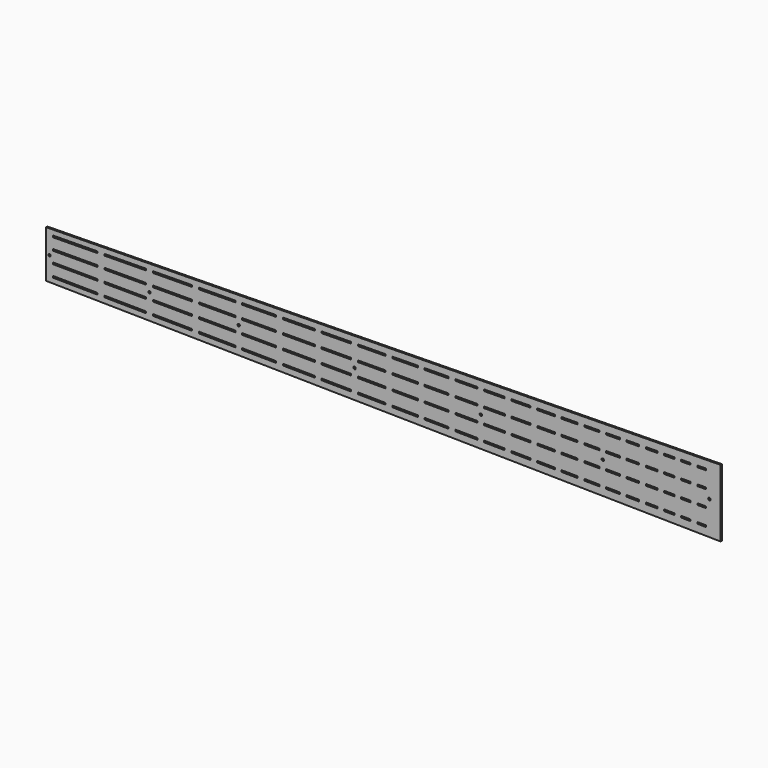
from build123d import *

# Parameters (mm, degrees)
F2_DEPTH = 1.524
F4_DEPTH = 1.525
F5_R     = 1.1303
F6_DEPTH = 979
F7_DEPTH = 1.525


# Not quite as in the source:
# - an extrude ends at something that could not be found from the text; its depth is read off the source's solid


with BuildPart() as f2:
    # F1 (on Front) → F2 (new body)
    with BuildSketch(Plane.XZ):
        Polygon((0, 44.45), (0, 0), (635, -9.525), (635, 53.975), align=None)
    extrude(amount=F2_DEPTH)

    # F0 (on Front) → F4 (cut, through all)
    with BuildSketch(Plane.XZ):
        Polygon((6.3580304305, 6.2480541955), (6.3496125138, 5.4861006938), (6.341194597, 4.7241471921), (48.4590379481, 4.2588373038), (48.4674558648, 5.0207908055), (48.4758737815, 5.7827443071), align=None)
        Polygon((54.8254862953, 5.7125950009), (54.8170683786, 4.9506414993), (54.8086504618, 4.1886879976), (94.2054562647, 3.7534396124), (94.2138741814, 4.515393114), (94.2222920981, 5.2773466157), align=None)
        Polygon((100.5719046119, 5.2071973095), (100.5634866952, 4.4452438078), (100.5550687784, 3.6832903062), (137.385412, 3.2763957093), (137.3938299168, 4.0383492109), (137.4022478336, 4.8003027126), align=None)
        Polygon((143.7518603473, 4.7301534064), (143.7434424306, 3.9681999047), (143.7350245139, 3.2062464031), (178.1336185335, 2.8262173069), (178.1420364502, 3.5881708085), (178.150454367, 4.3501243102), align=None)
        Polygon((184.5000668807, 4.279975004), (184.491648964, 3.5180215023), (184.4832310472, 2.7560680007), (216.6098321156, 2.4011394486), (216.6182500324, 3.1630929503), (216.6266679491, 3.9250464519), align=None)
        Polygon((222.9762804629, 3.8548971457), (222.9678625461, 3.0929436441), (222.9594446294, 2.3309901424), (252.9185419701, 2.0000077576), (252.9269598868, 2.7619612592), (252.9353778036, 3.5239147609), align=None)
        Polygon((259.2849903173, 3.4537654547), (259.2765724006, 2.691811953), (259.2681544838, 1.9298584514), (287.1901437394, 1.6213816475), (287.1985616562, 2.3833351492), (287.2069795729, 3.1452886508), align=None)
        Polygon((293.5565920867, 3.0751393446), (293.5481741699, 2.313185843), (293.5397562532, 1.5512323413), (319.5377621202, 1.2640113384), (319.5461800369, 2.0259648401), (319.5545979537, 2.7879183417), align=None)
        Polygon((325.9042104674, 2.7177690355), (325.8957925507, 1.9558155339), (325.887374634, 1.1938620322), (350.0702040724, 0.9266947518), (350.0786219892, 1.6886482534), (350.0870399059, 2.4506017551), align=None)
        Polygon((356.4366524197, 2.3804524489), (356.4282345029, 1.6184989472), (356.4198165862, 0.8565454456), (378.8893681778, 0.6083061315), (378.8977860945, 1.3702596332), (378.9062040113, 2.1322131349), align=None)
        Polygon((385.255816525, 2.0620638286), (385.2473986083, 1.300110327), (385.2389806915, 0.5381568253), (406.0902446394, 0.3077960441), (406.0986625561, 1.0697495457), (406.1070804729, 1.8317030474), align=None)
        Polygon((412.4566929866, 1.7615537412), (412.4482750699, 0.9996002395), (412.4398571532, 0.2376467379), (431.7652330186, 0.0241436767), (431.7736509354, 0.7860971784), (431.7820688521, 1.54805068), align=None)
        Polygon((438.1316813659, 1.4779013738), (438.1232634491, 0.7159478722), (438.1148455324, -0.0460056295), (455.998960951, -0.2435859206), (456.0073788678, 0.5183675811), (456.0157967845, 1.2803210827), align=None)
        Polygon((462.3654092983, 1.2101717765), (462.3569913815, 0.4482182749), (462.3485734648, -0.3137352268), (478.872601883, -0.4962895364), (478.8810197997, 0.2656639652), (478.8894377165, 1.0276174669), align=None)
        Polygon((485.2390502302, 0.9574681607), (485.2306323135, 0.195514659), (485.2222143967, -0.5664388426), (500.462147977, -0.7348067178), (500.4705658938, 0.0271467838), (500.4789838105, 0.7891002855), align=None)
        Polygon((506.8285963243, 0.7189509793), (506.8201784075, -0.0430025224), (506.8117604908, -0.804956024), (520.8401372066, -0.9599388504), (520.8485551233, -0.1979853487), (520.8569730401, 0.5639681529), align=None)
        Polygon((527.2065855538, 0.4938188467), (527.1981676371, -0.268134655), (527.1897497203, -1.0300881566), (540.0739262612, -1.172430078), (540.0823441779, -0.4104765763), (540.0907620946, 0.3514769253), align=None)
        Polygon((546.4403746084, 0.2813276191), (546.4319566917, -0.4806258825), (546.4235387749, -1.2425793842), (558.2291447357, -1.3730054638), (558.2375626524, -0.6110519622), (558.2459805692, 0.1509015395), align=None)
        Polygon((564.5955930829, 0.0807522333), (564.5871751662, -0.6812012684), (564.5787572494, -1.44315477), (575.3645138467, -1.5623137487), (575.3729317635, -0.8003602471), (575.3813496802, -0.0384067454), align=None)
        Polygon((581.730962194, -0.1085560516), (581.7225442772, -0.8705095533), (581.7141263605, -1.6324630549), (591.5387548107, -1.7410036734), (591.5471727275, -0.9790501718), (591.5555906442, -0.2170966701), align=None)
        Polygon((597.905203158, -0.2872459763), (597.8967852412, -1.049199478), (597.8883673245, -1.8111529796), (606.8045440132, -1.9096571966), (606.81296193, -1.1477036949), (606.8213798467, -0.3857501933), align=None)
        Polygon((613.1709923605, -0.4558994995), (613.1625744437, -1.2178530011), (613.154156527, -1.9798065028), (621.2145578395, -2.0688562768), (621.2229757563, -1.3069027752), (621.231393673, -0.5449492735), align=None)
        Polygon((6.3527629194, 17.4073617316), (6.3499569471, 16.6453668979), (6.3471509749, 15.8833720643), (48.4672789994, 15.7282687682), (48.4700849717, 16.4902636018), (48.4728909439, 17.2522584355), align=None)
        Polygon((54.8228478911, 17.2288753334), (54.8200419188, 16.4668804998), (54.8172359466, 15.7048856661), (94.2161788208, 15.559802871), (94.218984793, 16.3217977047), (94.2217907653, 17.0837925383), align=None)
        Polygon((100.5717477124, 17.0604094363), (100.5689417402, 16.2984146026), (100.5661357679, 15.5364197689), (137.3984768438, 15.4007882367), (137.401282816, 16.1627830703), (137.4040887883, 16.924777904), align=None)
        Polygon((143.7540457354, 16.9013948019), (143.7512397632, 16.1393999682), (143.7484337909, 15.3774051346), (178.148893755, 15.2507287692), (178.1516997272, 16.0127236028), (178.1545056995, 16.7747184365), align=None)
        Polygon((184.5044626466, 16.7513353344), (184.5016566744, 15.9893405008), (184.4988507021, 15.2273456671), (216.6271944712, 15.1090361498), (216.6300004434, 15.8710309834), (216.6328064157, 16.6330258171), align=None)
        Polygon((222.9827633628, 16.609642715), (222.9799573906, 15.8476478814), (222.9771514183, 15.0856530477), (252.9378738839, 14.9753255861), (252.9406798562, 15.7373204197), (252.9434858284, 16.4993152534), align=None)
        Polygon((259.2934427755, 16.4759321513), (259.2906368033, 15.7139373177), (259.2878308311, 14.951942484), (287.211334709, 14.8491168827), (287.2141406813, 15.6111117164), (287.2169466535, 16.37310655), align=None)
        Polygon((293.5669036007, 16.349723448), (293.5640976284, 15.5877286143), (293.5612916562, 14.8257337807), (319.5607077795, 14.7299934464), (319.5635137518, 15.49198828), (319.566319724, 16.2539831137), align=None)
        Polygon((325.9162766711, 16.2306000116), (325.9134706989, 15.468605178), (325.9106647266, 14.7066103443), (350.0948059576, 14.6175545842), (350.0976119298, 15.3795494178), (350.1004179021, 16.1415442515), align=None)
        Polygon((356.4503748492, 16.1181611494), (356.447568877, 15.3561663157), (356.4447629047, 14.5941714821), (378.9155333524, 14.5114250441), (378.9183393246, 15.2734198777), (378.9211452969, 16.0354147114), align=None)
        Polygon((385.271102244, 16.0120316093), (385.2682962718, 15.2500367757), (385.2654902995, 14.488041942), (406.1178853198, 14.4112550149), (406.120691292, 15.1732498486), (406.1234972643, 15.9352446822), align=None)
        Polygon((412.4734542114, 15.9118615802), (412.4706482392, 15.1498667465), (412.4678422669, 14.3878719129), (431.7942664333, 14.3167042258), (431.7970724056, 15.0786990595), (431.7998783778, 15.8406938931), align=None)
        Polygon((438.1498353249, 15.817310791), (438.1470293527, 15.0553159574), (438.1442233804, 14.2933211237), (456.0293089191, 14.2274610267), (456.0321148914, 14.9894558604), (456.0349208636, 15.751450694), align=None)
        Polygon((462.3848778108, 15.728067592), (462.3820718385, 14.9660727583), (462.3792658663, 14.2040779246), (478.9041906269, 14.1432264881), (478.9069965991, 14.9052213217), (478.9098025714, 15.6672161554), align=None)
        Polygon((485.2597595185, 15.6438330533), (485.2569535463, 14.8818382197), (485.254147574, 14.119843386), (500.4949078413, 14.063720761), (500.4977138136, 14.8257155946), (500.5005197858, 15.5877104283), align=None)
        Polygon((506.850476733, 15.5643273262), (506.8476707607, 14.8023324925), (506.8448647885, 14.0403376589), (520.8740024706, 13.9886767168), (520.8768084428, 14.7506715504), (520.8796144151, 15.5126663841), align=None)
        Polygon((527.2295713622, 15.489283282), (527.22676539, 14.7272884483), (527.2239594177, 13.9652936147), (540.1088348579, 13.9178463076), (540.1116408302, 14.6798411412), (540.1144468024, 15.4418359749), align=None)
        Polygon((546.4644037496, 15.4184528728), (546.4615977773, 14.6564580392), (546.4587918051, 13.8944632055), (558.2650381585, 13.8509878456), (558.2678441307, 14.6129826793), (558.270650103, 15.3749775129), align=None)
        Polygon((564.6206070501, 15.3515944109), (564.6178010778, 14.5895995772), (564.6149951056, 13.8276047435), (575.4013367739, 13.787885084), (575.4041427462, 14.5498799176), (575.4069487184, 15.3118747513), align=None)
        Polygon((581.7569056656, 15.2884916492), (581.7540996933, 14.5264968156), (581.7512937211, 13.7645019819), (591.5764551063, 13.7283217758), (591.5792610785, 14.4903166094), (591.5820670508, 15.2523114431), align=None)
        Polygon((597.9320239979, 15.228928341), (597.9292180256, 14.4669335073), (597.9264120534, 13.7049386737), (606.8430723982, 13.6721039347), (606.8458783705, 14.4340987684), (606.8486843427, 15.196093602), align=None)
        Polygon((613.1986412899, 15.1727104999), (613.1958353176, 14.4107156663), (613.1930293454, 13.6487208326), (621.2538678927, 13.6190375746), (621.2566738649, 14.3810324083), (621.2594798372, 15.1430272419), align=None)
        Polygon((6.3471509749, 28.5666279357), (6.3499569471, 27.8046331021), (6.3527629194, 27.0426382684), (48.4728909439, 27.1977415645), (48.4700849717, 27.9597363982), (48.4672789994, 28.7217312318), align=None)
        Polygon((54.8172359466, 28.7451143339), (54.8200419188, 27.9831195002), (54.8228478911, 27.2211246666), (94.2217907653, 27.3662074617), (94.218984793, 28.1282022953), (94.2161788208, 28.890197129), align=None)
        Polygon((100.5661357679, 28.9135802311), (100.5689417402, 28.1515853974), (100.5717477124, 27.3895905637), (137.4040887883, 27.525222096), (137.401282816, 28.2872169297), (137.3984768438, 29.0492117633), align=None)
        Polygon((143.7484337909, 29.0725948654), (143.7512397632, 28.3106000318), (143.7540457354, 27.5486051981), (178.1545056995, 27.6752815635), (178.1516997272, 28.4372763972), (178.148893755, 29.1992712308), align=None)
        Polygon((184.4988507021, 29.2226543329), (184.5016566744, 28.4606594992), (184.5044626466, 27.6986646656), (216.6328064157, 27.8169741829), (216.6300004434, 28.5789690166), (216.6271944712, 29.3409638502), align=None)
        Polygon((222.9771514183, 29.3643469523), (222.9799573906, 28.6023521186), (222.9827633628, 27.840357285), (252.9434858284, 27.9506847466), (252.9406798562, 28.7126795803), (252.9378738839, 29.4746744139), align=None)
        Polygon((259.2878308311, 29.498057516), (259.2906368033, 28.7360626823), (259.2934427755, 27.9740678487), (287.2169466535, 28.07689345), (287.2141406813, 28.8388882836), (287.211334709, 29.6008831173), align=None)
        Polygon((293.5612916562, 29.6242662193), (293.5640976284, 28.8622713857), (293.5669036007, 28.100276552), (319.566319724, 28.1960168863), (319.5635137518, 28.95801172), (319.5607077795, 29.7200065536), align=None)
        Polygon((325.9106647266, 29.7433896557), (325.9134706989, 28.981394822), (325.9162766711, 28.2193999884), (350.1004179021, 28.3084557485), (350.0976119298, 29.0704505822), (350.0948059576, 29.8324454158), align=None)
        Polygon((356.4447629047, 29.8558285179), (356.447568877, 29.0938336843), (356.4503748492, 28.3318388506), (378.9211452969, 28.4145852886), (378.9183393246, 29.1765801223), (378.9155333524, 29.9385749559), align=None)
        Polygon((385.2654902995, 29.961958058), (385.2682962718, 29.1999632243), (385.271102244, 28.4379683907), (406.1234972643, 28.5147553178), (406.120691292, 29.2767501514), (406.1178853198, 30.0387449851), align=None)
        Polygon((412.4678422669, 30.0621280871), (412.4706482392, 29.3001332535), (412.4734542114, 28.5381384198), (431.7998783778, 28.6093061069), (431.7970724056, 29.3713009405), (431.7942664333, 30.1332957742), align=None)
        Polygon((438.1442233804, 30.1566788763), (438.1470293527, 29.3946840426), (438.1498353249, 28.632689209), (456.0349208636, 28.698549306), (456.0321148914, 29.4605441396), (456.0293089191, 30.2225389733), align=None)
        Polygon((462.3792658663, 30.2459220754), (462.3820718385, 29.4839272417), (462.3848778108, 28.721932408), (478.9098025714, 28.7827838446), (478.9069965991, 29.5447786783), (478.9041906269, 30.3067735119), align=None)
        Polygon((485.254147574, 30.330156614), (485.2569535463, 29.5681617803), (485.2597595185, 28.8061669467), (500.5005197858, 28.8622895717), (500.4977138136, 29.6242844054), (500.4949078413, 30.386279239), align=None)
        Polygon((506.8448647885, 30.4096623411), (506.8476707607, 29.6476675075), (506.850476733, 28.8856726738), (520.8796144151, 28.9373336159), (520.8768084428, 29.6993284496), (520.8740024706, 30.4613232832), align=None)
        Polygon((527.2239594177, 30.4847063853), (527.22676539, 29.7227115517), (527.2295713622, 28.960716718), (540.1144468024, 29.0081640251), (540.1116408302, 29.7701588588), (540.1088348579, 30.5321536924), align=None)
        Polygon((546.4587918051, 30.5555367945), (546.4615977773, 29.7935419608), (546.4644037496, 29.0315471272), (558.270650103, 29.0750224871), (558.2678441307, 29.8370173207), (558.2650381585, 30.5990121544), align=None)
        Polygon((564.6149951056, 30.6223952565), (564.6178010778, 29.8604004228), (564.6206070501, 29.0984055891), (575.4069487184, 29.1381252487), (575.4041427462, 29.9001200824), (575.4013367739, 30.662114916), align=None)
        Polygon((581.7512937211, 30.6854980181), (581.7540996933, 29.9235031844), (581.7569056656, 29.1615083508), (591.5820670508, 29.1976885569), (591.5792610785, 29.9596833906), (591.5764551063, 30.7216782242), align=None)
        Polygon((597.9264120534, 30.7450613263), (597.9292180256, 29.9830664927), (597.9320239979, 29.221071659), (606.8486843427, 29.253906398), (606.8458783705, 30.0159012316), (606.8430723982, 30.7778960653), align=None)
        Polygon((613.1930293454, 30.8012791674), (613.1958353176, 30.0392843337), (613.1986412899, 29.2772895001), (621.2594798372, 29.3069727581), (621.2566738649, 30.0689675917), (621.2538678927, 30.8309624254), align=None)
        Polygon((6.341194597, 39.7258528079), (6.3496125138, 38.9638993062), (6.3580304305, 38.2019458046), (48.4758737815, 38.6672556929), (48.4674558648, 39.4292091945), (48.4590379481, 40.1911626962), align=None)
        Polygon((54.8086504618, 40.2613120024), (54.8170683786, 39.4993585007), (54.8254862953, 38.7374049991), (94.2222920981, 39.1726533843), (94.2138741814, 39.934606886), (94.2054562647, 40.6965603876), align=None)
        Polygon((100.5550687784, 40.7667096938), (100.5634866952, 40.0047561922), (100.5719046119, 39.2428026905), (137.4022478336, 39.6496972874), (137.3938299168, 40.4116507891), (137.385412, 41.1736042907), align=None)
        Polygon((143.7350245139, 41.2437535969), (143.7434424306, 40.4818000953), (143.7518603473, 39.7198465936), (178.150454367, 40.0998756898), (178.1420364502, 40.8618291915), (178.1336185335, 41.6237826931), align=None)
        Polygon((184.4832310472, 41.6939319993), (184.491648964, 40.9319784977), (184.5000668807, 40.170024996), (216.6266679491, 40.5249535481), (216.6182500324, 41.2869070497), (216.6098321156, 42.0488605514), align=None)
        Polygon((222.9594446294, 42.1190098576), (222.9678625461, 41.3570563559), (222.9762804629, 40.5951028543), (252.9353778036, 40.9260852391), (252.9269598868, 41.6880387408), (252.9185419701, 42.4499922424), align=None)
        Polygon((259.2681544838, 42.5201415486), (259.2765724006, 41.758188047), (259.2849903173, 40.9962345453), (287.2069795729, 41.3047113492), (287.1985616562, 42.0666648508), (287.1901437394, 42.8286183525), align=None)
        Polygon((293.5397562532, 42.8987676587), (293.5481741699, 42.136814157), (293.5565920867, 41.3748606554), (319.5545979537, 41.6620816583), (319.5461800369, 42.4240351599), (319.5377621202, 43.1859886616), align=None)
        Polygon((325.887374634, 43.2561379678), (325.8957925507, 42.4941844661), (325.9042104674, 41.7322309645), (350.0870399059, 41.9993982449), (350.0786219892, 42.7613517466), (350.0702040724, 43.5233052482), align=None)
        Polygon((356.4198165862, 43.5934545544), (356.4282345029, 42.8315010528), (356.4366524197, 42.0695475511), (378.9062040113, 42.3177868652), (378.8977860945, 43.0797403668), (378.8893681778, 43.8416938685), align=None)
        Polygon((385.2389806915, 43.9118431747), (385.2473986083, 43.149889673), (385.255816525, 42.3879361714), (406.1070804729, 42.6182969526), (406.0986625561, 43.3802504543), (406.0902446394, 44.1422039559), align=None)
        Polygon((412.4398571532, 44.2123532621), (412.4482750699, 43.4503997605), (412.4566929866, 42.6884462588), (431.7820688521, 42.90194932), (431.7736509354, 43.6639028216), (431.7652330186, 44.4258563233), align=None)
        Polygon((438.1148455324, 44.4960056295), (438.1232634491, 43.7340521278), (438.1316813659, 42.9720986262), (456.0157967845, 43.1696789173), (456.0073788678, 43.9316324189), (455.998960951, 44.6935859206), align=None)
        Polygon((462.3485734648, 44.7637352268), (462.3569913815, 44.0017817251), (462.3654092983, 43.2398282235), (478.8894377165, 43.4223825331), (478.8810197997, 44.1843360348), (478.872601883, 44.9462895364), align=None)
        Polygon((485.2222143967, 45.0164388426), (485.2306323135, 44.254485341), (485.2390502302, 43.4925318393), (500.4789838105, 43.6608997145), (500.4705658938, 44.4228532162), (500.462147977, 45.1848067178), align=None)
        Polygon((506.8117604908, 45.254956024), (506.8201784075, 44.4930025224), (506.8285963243, 43.7310490207), (520.8569730401, 43.8860318471), (520.8485551233, 44.6479853487), (520.8401372066, 45.4099388504), align=None)
        Polygon((527.1897497203, 45.4800881566), (527.1981676371, 44.718134655), (527.2065855538, 43.9561811533), (540.0907620946, 44.0985230747), (540.0823441779, 44.8604765763), (540.0739262612, 45.622430078), align=None)
        Polygon((546.4235387749, 45.6925793842), (546.4319566917, 44.9306258825), (546.4403746084, 44.1686723809), (558.2459805692, 44.2990984605), (558.2375626524, 45.0610519622), (558.2291447357, 45.8230054638), align=None)
        Polygon((564.5787572494, 45.89315477), (564.5871751662, 45.1312012684), (564.5955930829, 44.3692477667), (575.3813496802, 44.4884067454), (575.3729317635, 45.2503602471), (575.3645138467, 46.0123137487), align=None)
        Polygon((581.7141263605, 46.0824630549), (581.7225442772, 45.3205095533), (581.730962194, 44.5585560516), (591.5555906442, 44.6670966701), (591.5471727275, 45.4290501718), (591.5387548107, 46.1910036734), align=None)
        Polygon((597.8883673245, 46.2611529796), (597.8967852412, 45.499199478), (597.905203158, 44.7372459763), (606.8213798467, 44.8357501933), (606.81296193, 45.5977036949), (606.8045440132, 46.3596571966), align=None)
        Polygon((613.154156527, 46.4298065028), (613.1625744437, 45.6678530011), (613.1709923605, 44.9058994995), (621.231393673, 44.9949492735), (621.2229757563, 45.7569027752), (621.2145578395, 46.5188562768), align=None)
    extrude(amount=F4_DEPTH, mode=Mode.SUBTRACT)

    # F5 (on face) → F6 (cut, through all)
    with BuildSketch(Plane.XZ.offset(1.524)):
        with Locations((97.3946236, 22.225)):
            Circle(F5_R)
        with Locations((3.175, 22.225)):
            Circle(F5_R)
        with Locations((181.3279076, 22.225)):
            Circle(F5_R)
        with Locations((290.391088, 22.225)):
            Circle(F5_R)
        with Locations((409.2984448, 22.225)):
            Circle(F5_R)
        with Locations((524.05534, 22.225)):
            Circle(F5_R)
        with Locations((624.435886, 22.225)):
            Circle(F5_R)
    extrude(amount=F6_DEPTH, mode=Mode.SUBTRACT)

    # F5 (on face) → F7 (cut, through all)
    with BuildSketch(Plane.XZ.offset(1.524)):
        with Locations((97.3946236, 22.225)):
            Circle(F5_R)
        with Locations((3.175, 22.225)):
            Circle(F5_R)
        with Locations((181.3279076, 22.225)):
            Circle(F5_R)
        with Locations((290.391088, 22.225)):
            Circle(F5_R)
        with Locations((409.2984448, 22.225)):
            Circle(F5_R)
        with Locations((524.05534, 22.225)):
            Circle(F5_R)
        with Locations((624.435886, 22.225)):
            Circle(F5_R)
    extrude(amount=-F7_DEPTH, mode=Mode.SUBTRACT)


solid = f2.part
